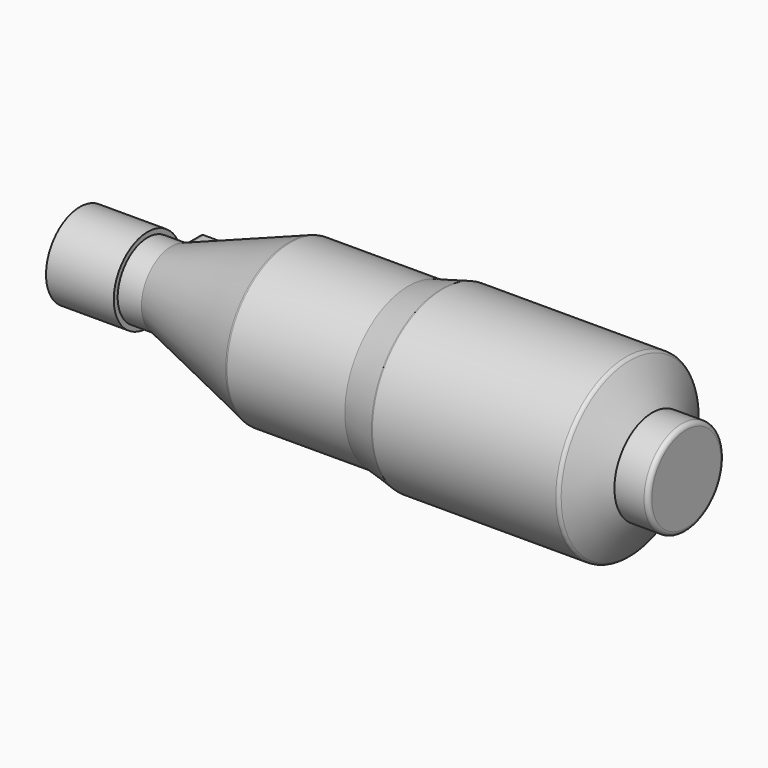
from build123d import *

# Parameters (mm, degrees)
F0_W     = 20
F0_H     = 11.0503323376
F0_H_2   = 1.4496676624
F0_W_2   = 35
F0_H_3   = 23.5
F0_W_3   = 10
F0_H_4   = 14
F2_DEPTH = 5
F3_DEPTH = 5
F4_DEPTH = 10
F6_R     = 1.27
F7_R     = 11.2300002947
F8_DEPTH = 15.24
F5_R     = 2.9447713958
F9_DEPTH = 1.778
F10_R    = 0.5518892204


with BuildPart() as f1:
    # F0 (on Top) → F1 (revolve)
    with BuildSketch(Plane.XY):
        with Locations((-45.1154029071, 5.5251661688)):
            Rectangle(F0_W, F0_H)
        with Locations((-45.1154029071, 11.7751661688)):
            Rectangle(F0_W, F0_H_2)
        Polygon((-35.1154029071, 11.0503323376), (-35.1154029071, 0), (-28.1154029071, 0), (-28.1154029071, 11.0503323376), (-34.2071130872, 11.0503323376), align=None)
        Polygon((-28.1154029071, 11.0503323376), (-28.1154029071, 0), (-17.1154029071, 0), (6.8845970929, 0), (6.8845970929, 23.5), (-17.1154029071, 14.9630850315), align=None)
        with Locations((24.3845970929, 11.75)):
            Rectangle(F0_W_2, F0_H_3)
        Polygon((41.8845970929, 23.5), (41.8845970929, 0), (51.8845970929, 0), (51.8845970929, 26), align=None)
        Polygon((51.8845970929, 26), (51.8845970929, 0), (106.8845970929, 0), (113.8845970929, 0), (113.8845970929, 14), (106.8845970929, 26), align=None)
        with Locations((118.8845970929, 7)):
            Rectangle(F0_W_3, F0_H_4)
    revolve(axis=Axis((34.3845970929, 0, 0), (1, 0, 0)))



with BuildPart() as f2:
    # F0 (on Top) → F2 (new body)
    with BuildSketch(Plane.XY):
        Polygon((-34.2071130872, 11.0503323376), (-28.1154029071, 11.0503323376), (-17.1154029071, 14.9630850315), (-26.2071130872, 18.0503323376), (-34.2071130872, 18.0503323376), align=None)
    extrude(amount=F2_DEPTH)


with BuildPart() as f1_1:
    add(f1.part)

    add(f2.part)  # F3 merges F2
    # F0 (on Top) → F3 (join)
    with BuildSketch(Plane.XY):
        Polygon((-34.2071130872, 11.0503323376), (-28.1154029071, 11.0503323376), (-17.1154029071, 14.9630850315), (-26.2071130872, 18.0503323376), (-34.2071130872, 18.0503323376), align=None)
    extrude(amount=-F3_DEPTH)

    # F4 (add): faces of the model
    f4_faces = [f1_1.faces().sort_by_distance(p)[0] for p in [
        (-31.1612579972, 11.0503323376, 2.5),
        (-31.1612579972, 11.0503323376, -2.5),
        (-22.6154029071, 13.0067086846, 2.5),
        (-22.6154029071, 13.0067086846, -2.5),
    ]]
    extrude(f4_faces, amount=F4_DEPTH, dir=(0, -1, 0))

    # F6
    f6_edges = [f1_1.edges().sort_by_distance(p)[0] for p in [
        (-34.207113, 13.952383, 5),
        (-34.207113, 13.952383, -5),
        (-34.661258, 11.050332, 0),
        (123.884597, -14, 0),
        (106.884597, -26, 0),
        (51.884597, -26, 0),
        (6.884597, -23.5, 0),
    ]]
    fillet(f6_edges, radius=F6_R)

    # F7 (on face) → F8 (cut)
    with BuildSketch(Plane(origin=(-55.1154029071, 0, 0), x_dir=(0, -1, 0), z_dir=(-1, 0, 0))):
        Circle(F7_R)
    extrude(amount=-F8_DEPTH, mode=Mode.SUBTRACT)

    # F5 (on face) → F9 (join)
    with BuildSketch(Plane(origin=(0, 18.0503323376, 0), x_dir=(-1, 0, 0), z_dir=(0, 1, 0))):
        with Locations((30.1491450518, 0)):
            Circle(F5_R)
    extrude(amount=F9_DEPTH)

    # F10
    f10_edges = [f1_1.edges().sort_by_distance(p)[0] for p in [
        (-27.204374, 19.828332, 0),
    ]]
    fillet(f10_edges, radius=F10_R)


solid = f1_1.part
